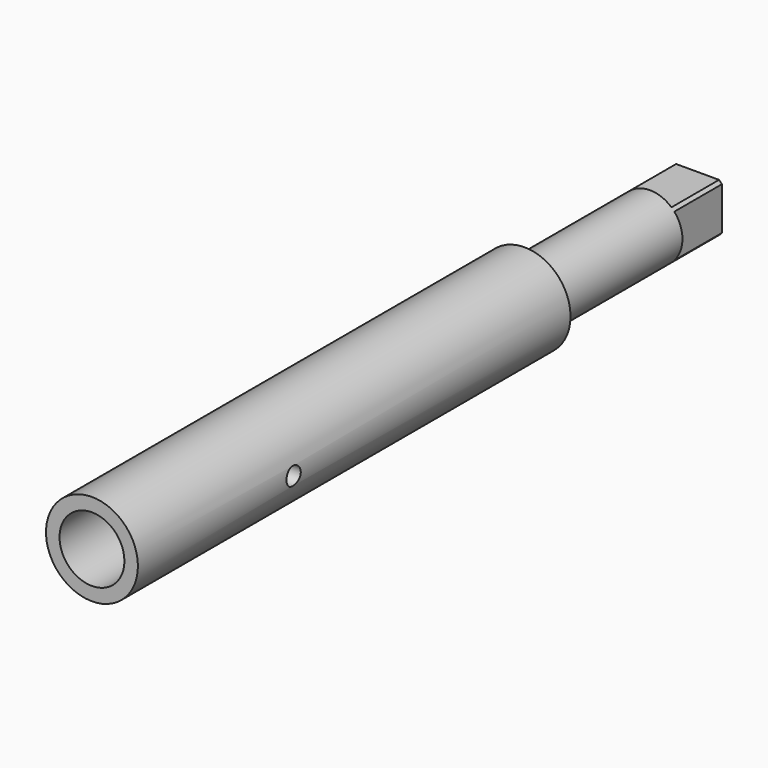
from build123d import *

# Parameters (mm, degrees)
F0_R      = 8.5
F1_DEPTH  = 140
F2_R      = 6
F3_DEPTH  = 30
F4_W      = 9
F4_H      = 9
F5_DEPTH  = 11
F6_SIZE   = 0.5
F7_SIZE   = 0.5
F8_SIZE   = 0.5
F9_R      = 1.65
F10_DEPTH = 25
F11_R     = 8.5
F11_R_2   = 6
F12_DEPTH = 40
F14_DEPTH = 11


# Not quite as in the source:
# - a pattern or mirror of a feature is missing from the dataset's text; its kind, count and spacing are read off the source's solid


with BuildPart() as f1:
    # F0 (on Front) → F1 (new body)
    with BuildSketch(Plane.XZ):
        Circle(F0_R)
    extrude(amount=F1_DEPTH)

    # F2 (on face) → F3 (cut)
    with BuildSketch(Plane.XZ.offset(140)):
        Circle(F2_R)
    extrude(amount=-F3_DEPTH, mode=Mode.SUBTRACT)

    # F4 (on face) → F5 (cut)
    with BuildSketch(Plane.XZ.offset(110)):
        Rectangle(F4_W, F4_H)
    extrude(amount=-F5_DEPTH, mode=Mode.SUBTRACT)

    # F6
    f6_edges = [f1.edges().sort_by_distance(p)[0] for p in [
        (-4.5, -104.5, -4.5),
    ]]
    chamfer(f6_edges, length=F6_SIZE)

    # F7
    f7_edges = [f1.edges().sort_by_distance(p)[0] for p in [
        (4.5, -104.5, -4.5),
    ]]
    chamfer(f7_edges, length=F7_SIZE)

    # F8
    f8_edges = [f1.edges().sort_by_distance(p)[0] for p in [
        (4.5, -104.5, 4.5),
        (-4.5, -104.5, 4.5),
    ]]
    chamfer(f8_edges, length=F8_SIZE)

    # F9 (on face) → F10 (cut)
    with BuildSketch(Plane.YZ.offset(-4.5)):
        with Locations((-104, 0)):
            Circle(F9_R)
    f10 = extrude(amount=-F10_DEPTH, mode=Mode.SUBTRACT)

    # F10_copies: F10 across plane
    add(f10.mirror(Plane(origin=(5.8e-05, 0, 0), x_dir=(1e-06, 1, 0), z_dir=(1, -1e-06, 0))), mode=Mode.SUBTRACT)

    # F11 (on face) → F12 (cut)
    with BuildSketch(Plane(origin=(0, 0, 0), x_dir=(-1, 0, 0), z_dir=(0, 1, 0))):
        Circle(F11_R)
        Circle(F11_R_2, mode=Mode.SUBTRACT)
    extrude(amount=-F12_DEPTH, mode=Mode.SUBTRACT)

    # F13 (on face) → F14 (cut)
    with BuildSketch(Plane(origin=(0, 0, 0), x_dir=(-1, 0, 0), z_dir=(0, 1, 0))):
        with BuildLine():
            Line((3.9686269666, -4.5), (-3.9686269666, -4.5))
            ThreePointArc((-3.9686269666, -4.5), (0, -6), (3.9686269666, -4.5))
        make_face()
        with BuildLine():
            ThreePointArc((-4.5, 3.9686269666), (-6, 0), (-4.5, -3.9686269666))
            Line((-4.5, -3.9686269666), (-4.5, 3.9686269666))
        make_face()
        with BuildLine():
            Line((-4.5, 4.5), (-4.5, 3.9686269666))
            ThreePointArc((-4.5, 3.9686269666), (-4.2426406871, 4.2426406871), (-3.9686269666, 4.5))
            Line((-3.9686269666, 4.5), (-4.5, 4.5))
        make_face()
        with BuildLine():
            Line((4.5, 3.9686269666), (4.5, -3.9686269666))
            ThreePointArc((4.5, -3.9686269666), (5.6124860802, -2.1213203436), (6, 0))
            ThreePointArc((6, 0), (5.6124860802, 2.1213203436), (4.5, 3.9686269666))
        make_face()
        with BuildLine():
            ThreePointArc((3.9686269666, 4.5), (0, 6), (-3.9686269666, 4.5))
            Line((-3.9686269666, 4.5), (3.9686269666, 4.5))
        make_face()
        with BuildLine():
            ThreePointArc((3.9686269666, 4.5), (4.2426406871, 4.2426406871), (4.5, 3.9686269666))
            Line((4.5, 3.9686269666), (4.5, 4.5))
            Line((4.5, 4.5), (3.9686269666, 4.5))
        make_face()
    extrude(amount=-F14_DEPTH, mode=Mode.SUBTRACT)


solid = f1.part
